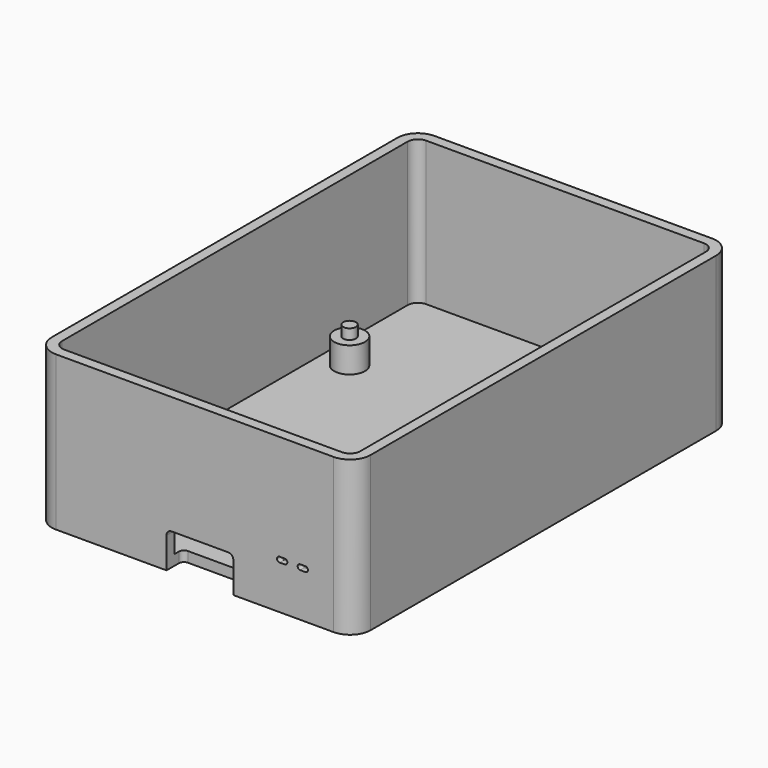
from build123d import *

# Parameters (mm, degrees)
F0_W          = 62
F0_H          = 92
F1_DEPTH      = 2
F2_W          = 62
F2_H          = 92
F2_W_2        = 58
F2_H_2        = 88
F2_R          = 3
F3_DEPTH      = 28
F4_DEPTH      = 23
F5_R          = 1.25
F6_DEPTH      = 2
F7_R          = 1.25
F8_DEPTH      = 2
F9_R          = 1.25
F10_DEPTH     = 2
F11_R         = 1.25
F12_DEPTH     = 2
F14_DEPTH     = 4
F15_R         = 1
F16_R         = 2
F17_R         = 4
F18_T1_DEPTH  = 1
F18_T3_DEPTH  = 1
F18_T6_ANGLE  = 180
F18_T8_ANGLE  = 180
F18_T10_ANGLE = 180
F18_T12_ANGLE = 180


# Not quite as in the source:
# - a fillet or chamfer that OpenCascade refuses, or shapes differently, is made with other operations: its cross-section is extruded or revolved along the edge and cut away or added


with BuildPart() as f1:
    # F0 (on Top) → F1 (new body)
    with BuildSketch(Plane.XY):
        with Locations((31, 46)):
            Rectangle(F0_W, F0_H)
    extrude(amount=F1_DEPTH)

    # F2 (on face) → F3 (join)
    with BuildSketch(Plane.XY.offset(2)):
        with Locations((31, 46)):
            Rectangle(F2_W, F2_H)
        with Locations((31, 46)):
            Rectangle(F2_W_2, F2_H_2, mode=Mode.SUBTRACT)
        with Locations((7.5, 67)):
            Circle(F2_R)
        with Locations((56.5, 67)):
            Circle(F2_R)
        with Locations((7.5, 9)):
            Circle(F2_R)
        with Locations((56.5, 9)):
            Circle(F2_R)
    extrude(amount=F3_DEPTH)

    # F4 (cut): faces of the model
    f4_faces = [f1.faces().sort_by_distance(p)[0] for p in [
        (7.5, 67, 30),
        (56.5, 67, 30),
        (56.5, 9, 30),
        (7.5, 9, 30),
    ]]
    extrude(f4_faces, amount=-F4_DEPTH, mode=Mode.SUBTRACT)

    # F5 (on face) → F6 (join)
    with BuildSketch(Plane.XY.offset(7)):
        with Locations((7.5, 9)):
            Circle(F5_R)
    extrude(amount=F6_DEPTH)

    # F7 (on face) → F8 (join)
    with BuildSketch(Plane.XY.offset(7)):
        with Locations((56.5, 9)):
            Circle(F7_R)
    extrude(amount=F8_DEPTH)

    # F9 (on face) → F10 (join)
    with BuildSketch(Plane.XY.offset(7)):
        with Locations((56.5, 67)):
            Circle(F9_R)
    extrude(amount=F10_DEPTH)

    # F11 (on face) → F12 (join)
    with BuildSketch(Plane.XY.offset(7)):
        with Locations((7.5, 67)):
            Circle(F11_R)
    extrude(amount=F12_DEPTH)

    # F13 (on face) → F14 (cut)
    with BuildSketch(Plane.XZ):
        with BuildLine():
            ThreePointArc((38.5, 6), (38.2071067812, 6.7071067812), (37.5, 7))
            Line((37.5, 7), (26.5, 7))
            ThreePointArc((26.5, 7), (25.7928932188, 6.7071067812), (25.5, 6))
            Line((25.5, 6), (25.5, 0))
            Line((25.5, 0), (38.5, 0))
            Line((38.5, 0), (38.5, 6))
        make_face()
        with BuildLine():
            Line((48.5, 9.5), (47.5, 9.5))
            ThreePointArc((47.5, 9.5), (47.1464466094, 9.3535533906), (47, 9))
            ThreePointArc((47, 9), (47.1464466094, 8.6464466094), (47.5, 8.5))
            Line((47.5, 8.5), (48.5, 8.5))
            ThreePointArc((48.5, 8.5), (48.8535533906, 8.6464466094), (49, 9))
            ThreePointArc((49, 9), (48.8535533906, 9.3535533906), (48.5, 9.5))
        make_face()
        with BuildLine():
            Line((52.5, 9.5), (51.5, 9.5))
            ThreePointArc((51.5, 9.5), (51.1464466094, 9.3535533906), (51, 9))
            ThreePointArc((51, 9), (51.1464466094, 8.6464466094), (51.5, 8.5))
            Line((51.5, 8.5), (52.5, 8.5))
            ThreePointArc((52.5, 8.5), (52.8535533906, 8.6464466094), (53, 9))
            ThreePointArc((53, 9), (52.8535533906, 9.3535533906), (52.5, 9.5))
        make_face()
    extrude(amount=-F14_DEPTH, mode=Mode.SUBTRACT)

    # F15
    f15_edges = [f1.edges().sort_by_distance(p)[0] for p in [
        (25.5, 4, 1),
        (38.5, 4, 1),
    ]]
    fillet(f15_edges, radius=F15_R)

    # F16
    f16_edges = [f1.edges().sort_by_distance(p)[0] for p in [
        (2, 90, 16),
        (60, 90, 16),
        (60, 2, 16),
        (2, 2, 16),
    ]]
    fillet(f16_edges, radius=F16_R)

    # F17
    f17_edges = [f1.edges().sort_by_distance(p)[0] for p in [
        (0, 92, 15),
        (62, 92, 15),
        (62, 0, 15),
        (0, 0, 15),
    ]]
    fillet(f17_edges, radius=F17_R)

    # F18: chamfer of 1 x 0.3639702343 on 8 edges, made by hand

    # F18_s2 → F18_t1 (cut)
    with BuildSketch(Plane.YZ.offset(51.5)):
        Polygon((2, 9.8639702343), (1, 9.5), (2, 9.5), align=None)
        Polygon((2, 8.1360297657), (1, 8.5), (2, 8.5), align=None)
    extrude(amount=F18_T1_DEPTH, mode=Mode.SUBTRACT)

    # F18_s4 → F18_t3 (cut)
    with BuildSketch(Plane.YZ.offset(47.5)):
        Polygon((2, 9.8639702343), (1, 9.5), (2, 9.5), align=None)
        Polygon((2, 8.1360297657), (1, 8.5), (2, 8.5), align=None)
    extrude(amount=F18_T3_DEPTH, mode=Mode.SUBTRACT)

    # F18_s5 → F18_t6 (revolve, cut)
    with BuildSketch(Plane.YZ.offset(51.5)):
        Polygon((2, 9.8639702343), (1, 9.5), (2, 9.5), align=None)
    revolve(axis=Axis((51.5, 2, 9), (0, -1, 0)), revolution_arc=F18_T6_ANGLE, mode=Mode.SUBTRACT)

    # F18_s7 → F18_t8 (revolve, cut)
    with BuildSketch(Plane.YZ.offset(47.5)):
        Polygon((2, 9.8639702343), (1, 9.5), (2, 9.5), align=None)
    revolve(axis=Axis((47.5, 2, 9), (0, -1, 0)), revolution_arc=F18_T8_ANGLE, mode=Mode.SUBTRACT)

    # F18_s9 → F18_t10 (revolve, cut)
    with BuildSketch(Plane.YZ.offset(52.5)):
        Polygon((2, 8.1360297657), (1, 8.5), (2, 8.5), align=None)
    revolve(axis=Axis((52.5, 2, 9), (0, -1, 0)), revolution_arc=F18_T10_ANGLE, mode=Mode.SUBTRACT)

    # F18_s11 → F18_t12 (revolve, cut)
    with BuildSketch(Plane.YZ.offset(48.5)):
        Polygon((2, 8.1360297657), (1, 8.5), (2, 8.5), align=None)
    revolve(axis=Axis((48.5, 2, 9), (0, -1, 0)), revolution_arc=F18_T12_ANGLE, mode=Mode.SUBTRACT)


solid = f1.part
